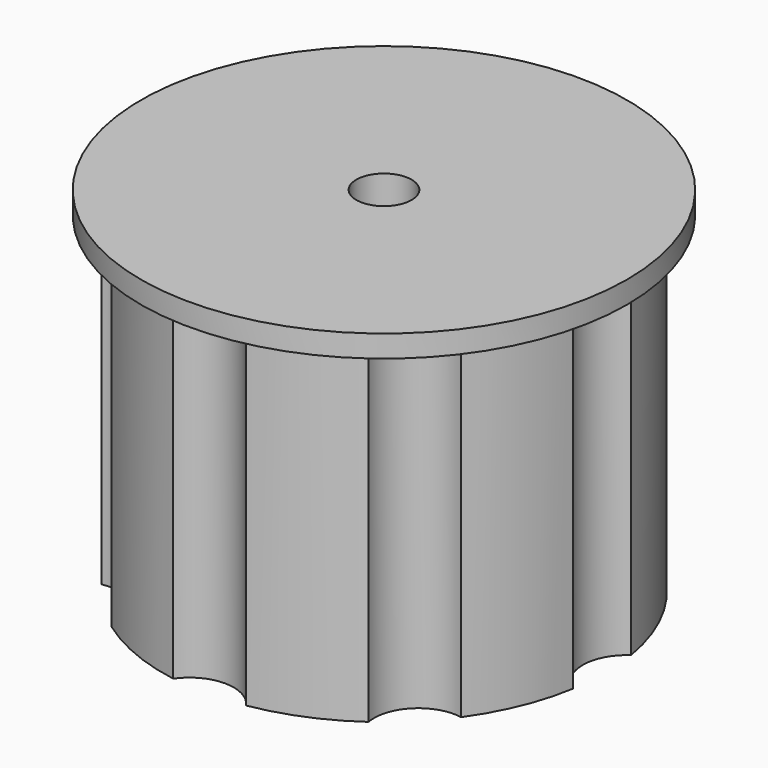
from build123d import *

# Parameters (mm, degrees)
F0_R            = 25.4
F1_DEPTH        = 19.05
F2_R            = 27.94
F2_R_2          = 25.4
F3_DEPTH        = 2.54
F4_R            = 22.352
F5_DEPTH        = 2.54
F6_R            = 3.175
F7_DEPTH        = 38.101
F9_DEPTH        = 38.1
F9_COPIES_COUNT = 8


# Not quite as in the source:
# - a pattern or mirror of a feature is missing from the dataset's text; its kind, count and spacing are read off the source's solid


with BuildPart() as f1:
    # F0 (on Top) → F1 (new body, symmetric)
    with BuildSketch(Plane.XY):
        Circle(F0_R)
    extrude(amount=F1_DEPTH, both=True)

    # F2 (on face) → F3 (join)
    with BuildSketch(Plane.XY.offset(19.05)):
        Circle(F2_R)
        Circle(F2_R_2, mode=Mode.SUBTRACT)
        Circle(F2_R_2)
    extrude(amount=F3_DEPTH)

    # F4 (on face) → F5 (cut)
    with BuildSketch(Plane(origin=(0, 0, -19.05), x_dir=(1, 0, 0), z_dir=(0, 0, -1))):
        Circle(F4_R)
    extrude(amount=-F5_DEPTH, mode=Mode.SUBTRACT)

    # F6 (on face) → F7 (cut, through all)
    with BuildSketch(Plane(origin=(0, 0, -16.51), x_dir=(1, 0, 0), z_dir=(0, 0, -1))):
        Circle(F6_R)
    extrude(amount=-F7_DEPTH, mode=Mode.SUBTRACT)

    # F8 (on face) → F9 (cut, through all)
    with BuildSketch(Plane(origin=(0, 0, -19.05), x_dir=(1, 0, 0), z_dir=(0, 0, -1))):
        with BuildLine():
            ThreePointArc((4.1803474687, 25.0536363636), (0, 25.4), (-4.1803474687, 25.0536363636))
            ThreePointArc((-4.1803474687, 25.0536363636), (0, 22.86), (4.1803474687, 25.0536363636))
        make_face()
    f9 = extrude(amount=-F9_DEPTH, mode=Mode.SUBTRACT)

    # F9_copies: F9 ×8 about axis
    f9_copies_axis = Axis((0, 0, 0), (0, 0, 1))
    for i in range(1, F9_COPIES_COUNT):
        add(f9.rotate(f9_copies_axis, i * 360 / F9_COPIES_COUNT), mode=Mode.SUBTRACT)


solid = f1.part
